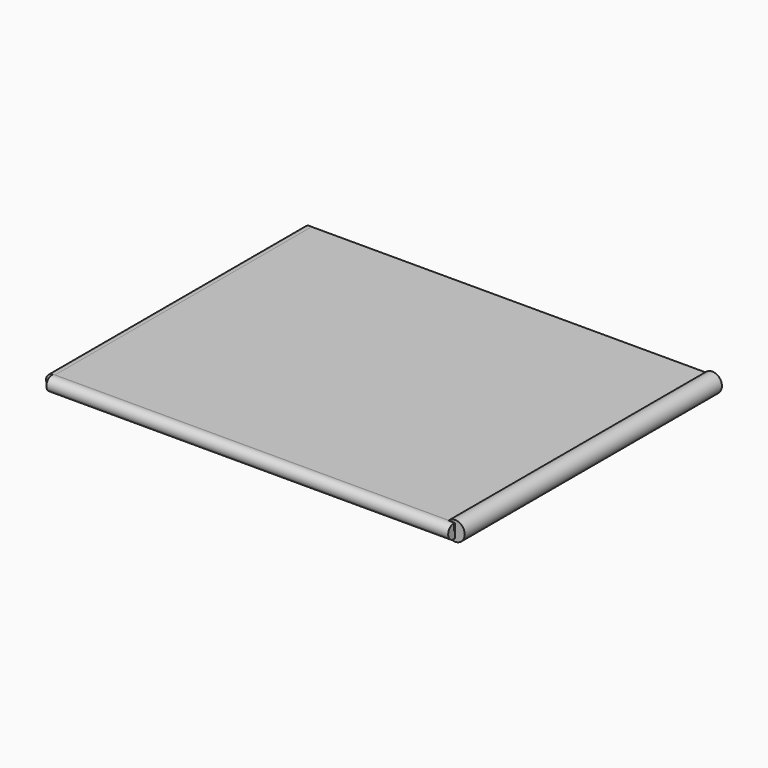
from build123d import *

# Parameters (mm, degrees)
F2_R      = 25.9962792711
F3_DEPTH  = 1219.2
F4_R      = 26.4847844062
F5_DEPTH  = 1524
F6_R      = 36.4583411444
F7_DEPTH  = 1219.2
F8_W      = 1525.4385471344
F8_H      = 1222.8087186813
F9_DEPTH  = 25.4
F15_DEPTH = 27.77983


# Not quite as in the source:
# - the program builds the solid bodies; features that only make, move or delete a surface that nothing else refers to are left out


with BuildPart() as f3:
    # F2 (on Front) → F3 (new body)
    with BuildSketch(Plane.XZ):
        Circle(F2_R)
    extrude(amount=F3_DEPTH)

    # F4 (on Right) → F5 (join)
    with BuildSketch(Plane.YZ):
        with Locations((-1223.8247394562, 0)):
            Circle(F4_R)
    extrude(amount=F5_DEPTH)

    # F6 (on Front) → F7 (join)
    with BuildSketch(Plane.XZ):
        with Locations((1525.4992246628, 0)):
            Circle(F6_R)
    extrude(amount=F7_DEPTH)

    # F8 (on Top) → F9 (join)
    with BuildSketch(Plane.XY):
        with Locations((762.7192735672, -611.4043593407)):
            Rectangle(F8_W, F8_H)
    extrude(amount=F9_DEPTH)

    # F15 (add): a face of the model
    f15_faces = [f3.faces().sort_by_distance(p)[0] for p in [
        (752.4403971283, -608.161243113, 25.4),
    ]]
    extrude(f15_faces, amount=-F15_DEPTH)


solid = f3.part
